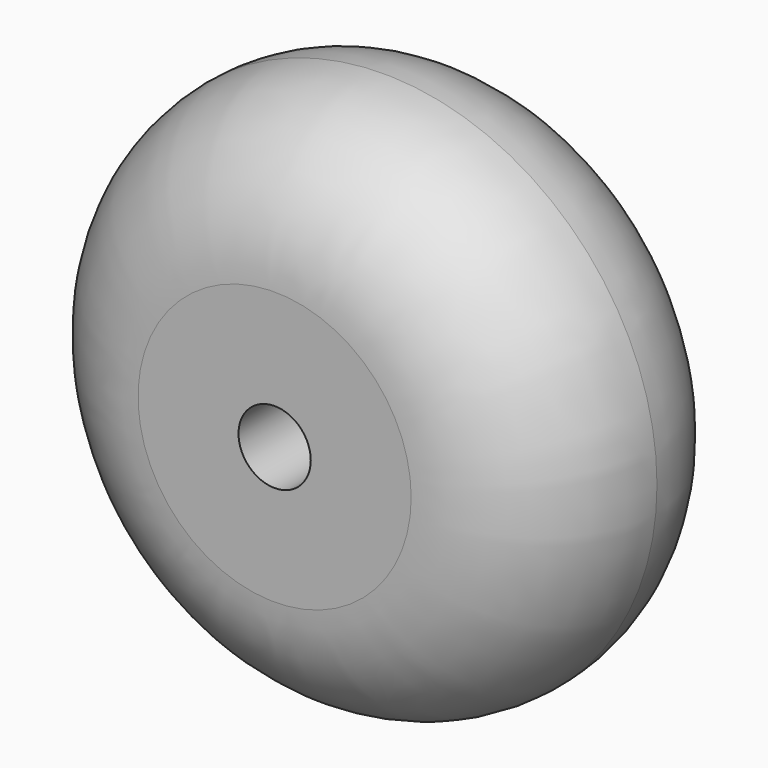
from build123d import *

# Parameters (mm, degrees)
F0_R     = 12
F0_R_2   = 1.5875
F1_DEPTH = 12
F2_R     = 5.99999


# Not quite as in the source:
# - a fillet or chamfer is up to 0.001 mm smaller than in the source, because OpenCascade refuses the exact size


with BuildPart() as f1:
    # F0 (on Front) → F1 (new body)
    with BuildSketch(Plane.XZ):
        Circle(F0_R)
        Circle(F0_R_2, mode=Mode.SUBTRACT)
    extrude(amount=F1_DEPTH)

    # F2 (radius 6 in the source; OpenCascade refuses exactly that, so slightly less here)
    f2_edges = [f1.edges().sort_by_distance(p)[0] for p in [
        (-12, -12, 0),
        (-12, 0, 0),
    ]]
    fillet(f2_edges, radius=F2_R)


solid = f1.part
